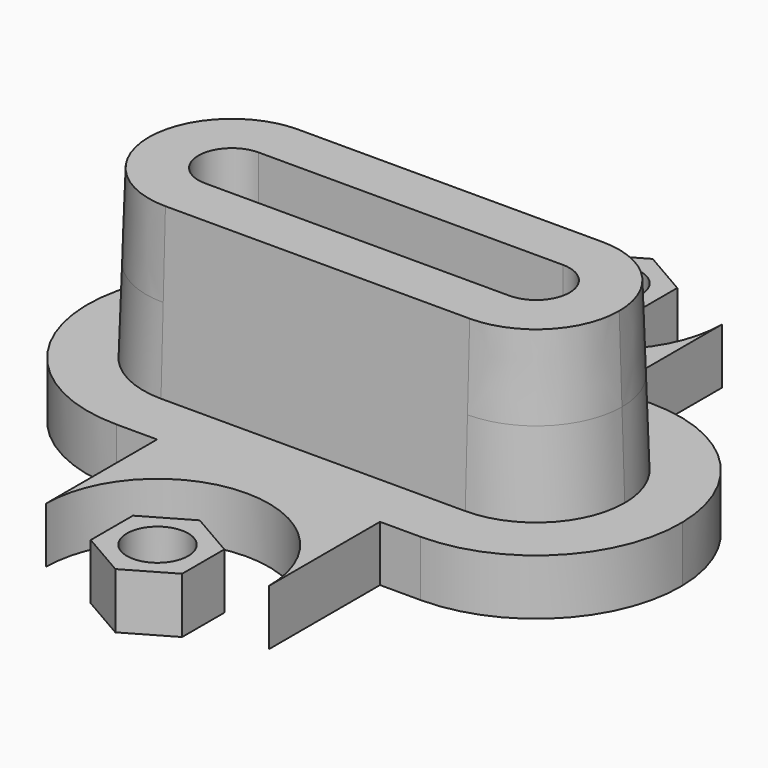
from build123d import *

# Parameters (mm, degrees)
F2_DEPTH      = 7.5
F2_TAPER      = 1.909
F2_DEPTH_BACK = 7.5
F2_TAPER_BACK = -1.909
F3_DEPTH      = 7.5
F3_DEPTH_BACK = 7.5
F5_DEPTH      = 5
F4_R          = 2.75


# Not quite as in the source:
# - a feature of the source that left no trace in its solid (it failed there, or was rolled back) is left out
# - a feature names something its author has since deleted; it is built from what else it names


with BuildPart() as f2:
    # F0 (on Top) → F2 (new body, two sides)
    with BuildSketch(Plane.XY) as f2_sk:
        with BuildLine():
            Line((13.65, 7.7), (-13.65, 7.7))
            ThreePointArc((-13.65, 7.7), (-19.0947222151, 5.4447222151), (-21.35, 0))
            ThreePointArc((-21.35, 0), (-19.0947222151, -5.4447222151), (-13.65, -7.7))
            Line((-13.65, -7.7), (13.65, -7.7))
            ThreePointArc((13.65, -7.7), (19.0947222151, -5.4447222151), (21.35, 0))
            ThreePointArc((21.35, 0), (19.0947222151, 5.4447222151), (13.65, 7.7))
        make_face()
    extrude(amount=F2_DEPTH, taper=F2_TAPER)
    extrude(f2_sk.sketch, amount=-F2_DEPTH_BACK, taper=F2_TAPER_BACK)

    # F1 (on Top) → F3 (cut, two sides)
    with BuildSketch(Plane.XY) as f3_sk:
        with BuildLine():
            Line((13.65, 3), (-13.65, 3))
            ThreePointArc((-13.65, 3), (-15.7713203436, 2.1213203436), (-16.65, 0))
            ThreePointArc((-16.65, 0), (-15.7713203436, -2.1213203436), (-13.65, -3))
            Line((-13.65, -3), (13.65, -3))
            ThreePointArc((13.65, -3), (15.7713203436, -2.1213203436), (16.65, 0))
            ThreePointArc((16.65, 0), (15.7713203436, 2.1213203436), (13.65, 3))
        make_face()
    extrude(amount=F3_DEPTH, mode=Mode.SUBTRACT)
    extrude(f3_sk.sketch, amount=-F3_DEPTH_BACK, mode=Mode.SUBTRACT)

    # F4 (on face) → F5 (join)
    with BuildSketch(Plane(origin=(0, 0, -7.5), x_dir=(1, 0, 0), z_dir=(0, 0, -1))):
        with BuildLine():
            Line((-10, 12.9499800244), (-13.65, 12.9499800244))
            ThreePointArc((-13.65, 12.9499800244), (-22.7251585222, 9.2381535184), (-26.597928487, 0.2305006046))
            ThreePointArc((-26.597928487, 0.2305006046), (-22.8881535184, -9.0751585222), (-13.65, -12.9499800244))
            Line((-13.65, -12.9499800244), (-10, -12.9499800244))
            Line((-10, -12.9499800244), (10, -12.9499800244))
            Line((10, -12.9499800244), (13.65, -12.9499800244))
            ThreePointArc((13.65, -12.9499800244), (22.7251585222, -9.2381535184), (26.597928487, -0.2305006046))
            ThreePointArc((26.597928487, -0.2305006046), (22.8881535184, 9.0751585222), (13.65, 12.9499800244))
            Line((13.65, 12.9499800244), (10, 12.9499800244))
            Line((10, 12.9499800244), (-10, 12.9499800244))
        make_face()
        with BuildLine():
            Line((13.65, -7.9499800244), (-13.65, -7.9499800244))
            ThreePointArc((-13.65, -7.9499800244), (-19.2714847855, -5.6214847855), (-21.5999800244, 0))
            ThreePointArc((-21.5999800244, 0), (-19.2714847855, 5.6214847855), (-13.65, 7.9499800244))
            Line((-13.65, 7.9499800244), (13.65, 7.9499800244))
            ThreePointArc((13.65, 7.9499800244), (19.2714847855, 5.6214847855), (21.5999800244, 0))
            ThreePointArc((21.5999800244, 0), (19.2714847855, -5.6214847855), (13.65, -7.9499800244))
        make_face(mode=Mode.SUBTRACT)
        with BuildLine():
            ThreePointArc((-21.5999800244, 0), (-19.2714847855, -5.6214847855), (-13.65, -7.9499800244))
            Line((-13.65, -7.9499800244), (13.65, -7.9499800244))
            ThreePointArc((13.65, -7.9499800244), (19.2714847855, -5.6214847855), (21.5999800244, 0))
            ThreePointArc((21.5999800244, 0), (19.2714847855, 5.6214847855), (13.65, 7.9499800244))
            Line((13.65, 7.9499800244), (-13.65, 7.9499800244))
            ThreePointArc((-13.65, 7.9499800244), (-19.2714847855, 5.6214847855), (-21.5999800244, 0))
        make_face()
        with BuildLine():
            ThreePointArc((13.65, 3), (16.65, 0), (13.65, -3))
            Line((13.65, -3), (-13.65, -3))
            ThreePointArc((-13.65, -3), (-16.65, 0), (-13.65, 3))
            Line((-13.65, 3), (13.65, 3))
        make_face(mode=Mode.SUBTRACT)
        with BuildLine():
            Line((-10, 25.4), (-10, 12.9499800244))
            Line((-10, 12.9499800244), (10, 12.9499800244))
            Line((10, 12.9499800244), (10, 25.4))
            ThreePointArc((10, 25.4), (0, 15.4), (-10, 25.4))
        make_face()
        with BuildLine():
            Line((10, -12.9499800244), (-10, -12.9499800244))
            Line((-10, -12.9499800244), (-10, -25.4))
            ThreePointArc((-10, -25.4), (0, -15.4), (10, -25.4))
            Line((10, -25.4), (10, -12.9499800244))
        make_face()
    extrude(amount=F5_DEPTH)


with BuildPart() as f5:
    # F4 (on face) → F5, piece 2 (new body)
    with BuildSketch(Plane(origin=(0, 0, -7.5), x_dir=(1, 0, 0), z_dir=(0, 0, -1))):
        Polygon((4.1, -23.0328638963), (0, -20.6657277926), (-4.1, -23.0328638963), (-4.1, -27.7671361037), (0, -30.1342722074), (4.1, -27.7671361037), align=None)
        with Locations((0, -25.4)):
            Circle(F4_R, mode=Mode.SUBTRACT)
    extrude(amount=F5_DEPTH)


with BuildPart() as f5b:
    # F4 (on face) → F5, piece 3 (new body)
    with BuildSketch(Plane(origin=(0, 0, -7.5), x_dir=(1, 0, 0), z_dir=(0, 0, -1))):
        Polygon((4.1, 23.0328638963), (4.1, 27.7671361037), (0, 30.1342722074), (-4.1, 27.7671361037), (-4.1, 23.0328638963), (0, 20.6657277926), align=None)
        with Locations((0, 25.4)):
            Circle(F4_R, mode=Mode.SUBTRACT)
    extrude(amount=F5_DEPTH)


solid = Compound([f2.part, f5.part, f5b.part])
